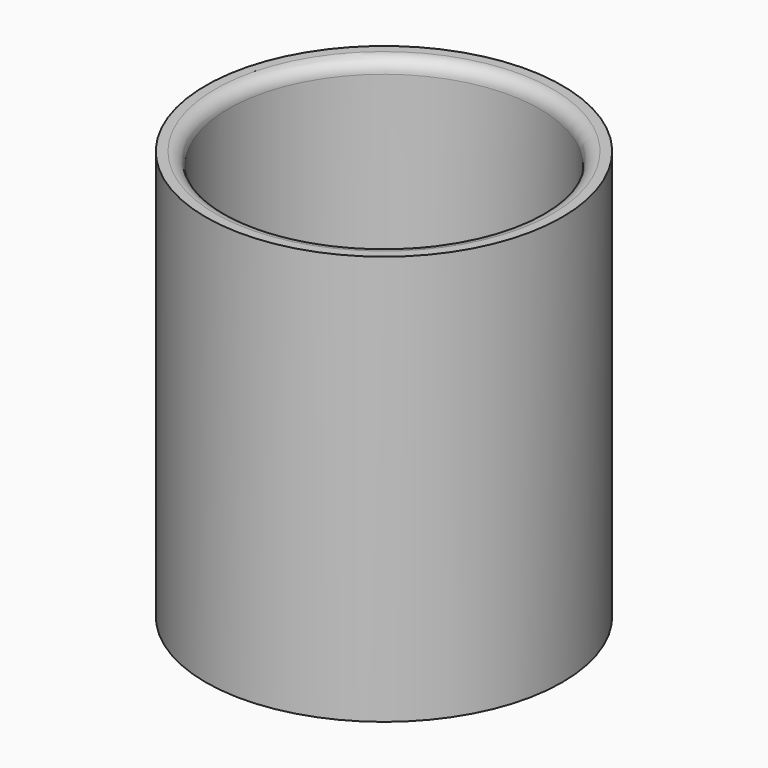
from build123d import *

# Parameters (mm, degrees)
F0_R          = 34.544
F0_R_2        = 30.1625
F1_DEPTH      = 39.6875
F1_DEPTH_BACK = 39.6875
F0_R_3        = 28.575
F2_DEPTH      = 2.38125
F2_DEPTH_BACK = 2.38125
F3_R          = 2.54


# Not quite as in the source:
# - a length typed as a fraction of an inch, garbled in the dataset ("3 / 203.2 mm" for 3/8 in), is restored


with BuildPart() as f1:
    # F0 (on Top) → F1 (new body, two sides)
    with BuildSketch(Plane.XY) as f1_sk:
        Circle(F0_R)
        Circle(F0_R_2, mode=Mode.SUBTRACT)
    extrude(amount=F1_DEPTH)
    extrude(f1_sk.sketch, amount=-F1_DEPTH_BACK)

    # F0 (on Top) → F2 (join, two sides)
    with BuildSketch(Plane.XY) as f2_sk:
        Circle(F0_R_2)
        Circle(F0_R_3, mode=Mode.SUBTRACT)
    extrude(amount=F2_DEPTH)
    extrude(f2_sk.sketch, amount=-F2_DEPTH_BACK)

    # F3
    f3_edges = [f1.edges().sort_by_distance(p)[0] for p in [
        (-30.1625, 0, 39.6875),
        (-30.1625, 0, -39.6875),
    ]]
    fillet(f3_edges, radius=F3_R)


solid = f1.part
